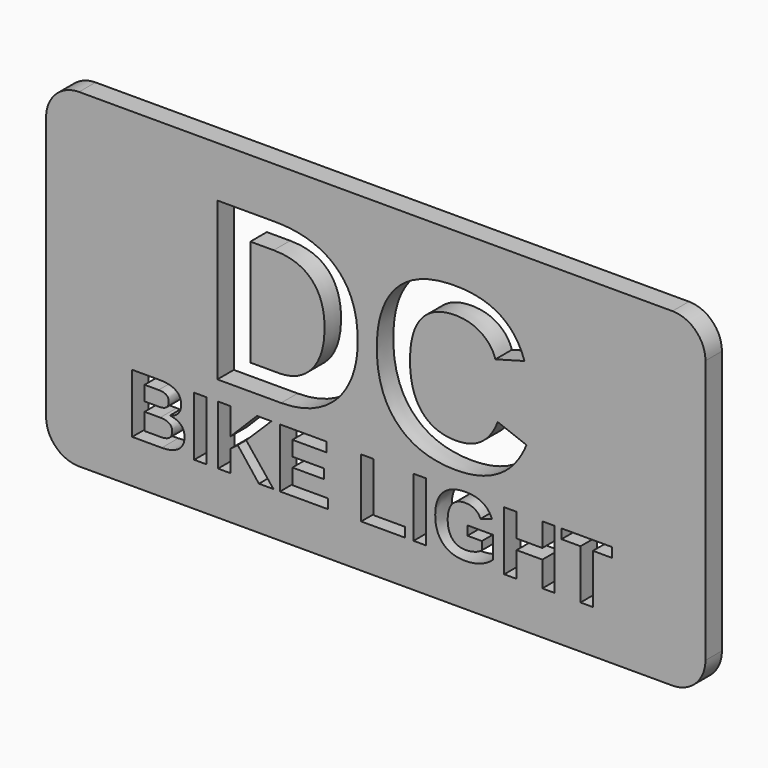
from build123d import *

# Parameters (mm, degrees)
F0_W           = 101.6
F0_H           = 50.8
F1_DEPTH       = 3.175
F2_R           = 5.08
F3_TEXT_SIZE   = 35.2777777778
F3_TEXT_SIZE_2 = 13.2291666667
F4_DEPTH       = 3.175


# Not quite as in the source:
# - Text() gives the source's letters only with a copy of the font that has no kerning and outlines rounded to 1/6400 em; it was checked with that copy


with BuildPart() as f1:
    # F0 (on Front) → F1 (new body)
    with BuildSketch(Plane.XZ):
        Rectangle(F0_W, F0_H)
    extrude(amount=F1_DEPTH)

    # F2
    f2_edges = [f1.edges().sort_by_distance(p)[0] for p in [
        (-50.8, -1.5875, 25.4),
        (50.8, -1.5875, 25.4),
        (50.8, -1.5875, -25.4),
        (-50.8, -1.5875, -25.4),
    ]]
    fillet(f2_edges, radius=F2_R)

    # F3 (on face) → F4 (cut, through all)
    with BuildSketch(Plane.XZ.offset(3.175)):
        with Locations((-26.7669255456, -6.6675)):
            Text('DC', F3_TEXT_SIZE, font='Arimo', font_style=FontStyle.BOLD, text_align=(TextAlign.LEFT, TextAlign.BOTTOM))
        with Locations((-38.4178939701, -18.7325)):
            Text('BIKE LIGHT', F3_TEXT_SIZE_2, font='Arimo', font_style=FontStyle.BOLD, text_align=(TextAlign.LEFT, TextAlign.BOTTOM))
    extrude(amount=-F4_DEPTH, mode=Mode.SUBTRACT)


solid = f1.part
